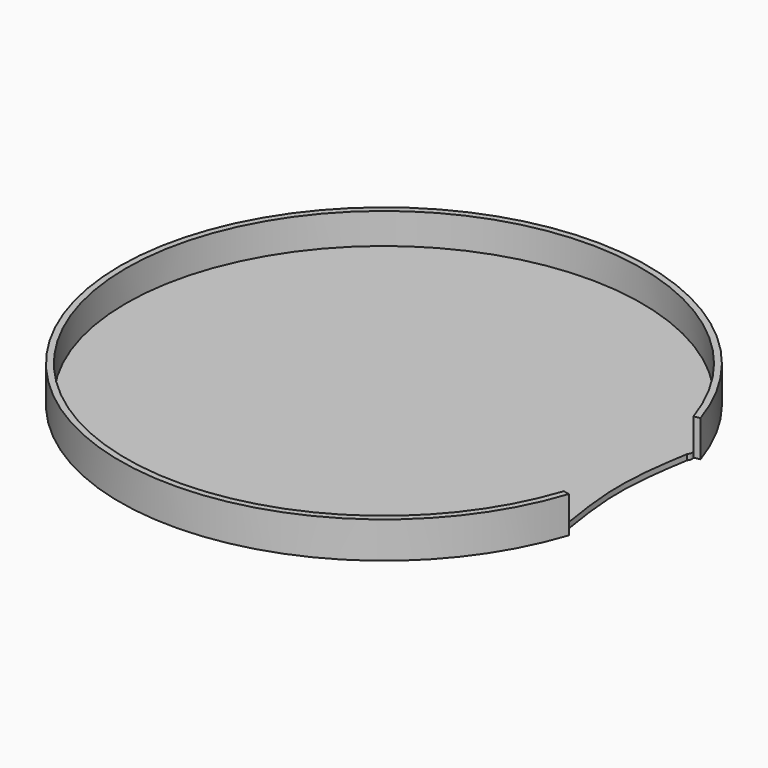
from build123d import *

# Parameters (mm, degrees)
F1_DEPTH    = 0.9
F2_DEPTH    = 5
F3_T1_DEPTH = 5.4053483188


# Not quite as in the source:
# - a fillet or chamfer that OpenCascade refuses, or shapes differently, is made with other operations: its cross-section is extruded or revolved along the edge and cut away or added


with BuildPart() as f1:
    # F0 (on Top) → F1 (new body)
    with BuildSketch(Plane.XY):
        with BuildLine():
            ThreePointArc((39.6825934579, 13.1351351897), (40.1749239484, 13.2423176115), (40.670911215, 13.3310532572))
            ThreePointArc((40.670911215, 13.3310532572), (-42.8, 0), (40.670911215, -13.3310532572))
            ThreePointArc((40.670911215, -13.3310532572), (40.1749239484, -13.2423176115), (39.6825934579, -13.1351351897))
            ThreePointArc((39.6825934579, -13.1351351897), (-41.8, 0), (39.6825934579, 13.1351351897))
        make_face()
        with BuildLine():
            ThreePointArc((39.5091459772, 12.0590331205), (39.7471474208, 12.1214723169), (39.9863317757, 12.179214717))
            ThreePointArc((39.9863317757, 12.179214717), (39.8373299552, 12.6580860339), (39.6825934579, 13.1351351897))
            add(Edge.make_bspline(
                [(39.5091459772, 12.0590331205), (39.5667025259, 12.4177338102), (39.6246479919, 12.7764345), (39.6825934579, 13.1351351897)],
                knots=[0.9590372671, 0.9590372671, 0.9590372671, 0.9590372671, 1, 1, 1, 1], degree=3))
        make_face()
        with BuildLine():
            ThreePointArc((39.6825934579, -13.1351351897), (39.8373299552, -12.6580860339), (39.9863317757, -12.179214717))
            ThreePointArc((39.9863317757, -12.179214717), (39.7471474208, -12.1214723169), (39.5091459772, -12.0590331205))
            add(Edge.make_bspline(
                [(39.6825934579, -13.1351351897), (39.6246479919, -12.7764345), (39.5667025259, -12.4177338102), (39.5091459772, -12.0590331205)],
                knots=[0, 0, 0, 0, 0.0409627329, 0.0409627329, 0.0409627329, 0.0409627329], degree=3))
        make_face()
        with BuildLine():
            add(Edge.make_bspline(
                [(39.5091459772, 12.0590331205), (39.5667025259, 12.4177338102), (39.6246479919, 12.7764345), (39.6825934579, 13.1351351897)],
                knots=[0.9590372671, 0.9590372671, 0.9590372671, 0.9590372671, 1, 1, 1, 1], degree=3))
            ThreePointArc((39.6825934579, 13.1351351897), (29.3, 0), (39.6825934579, -13.1351351897))
            add(Edge.make_bspline(
                [(39.6825934579, -13.1351351897), (39.6246479919, -12.7764345), (39.5667025259, -12.4177338102), (39.5091459772, -12.0590331205)],
                knots=[0, 0, 0, 0, 0.0409627329, 0.0409627329, 0.0409627329, 0.0409627329], degree=3))
            ThreePointArc((39.5091459772, -12.0590331205), (30.3, 0), (39.5091459772, 12.0590331205))
        make_face()
        with BuildLine():
            ThreePointArc((39.6825934579, -13.1351351897), (29.3, 0), (39.6825934579, 13.1351351897))
            ThreePointArc((39.6825934579, 13.1351351897), (-41.8, 0), (39.6825934579, -13.1351351897))
        make_face()
        with BuildLine():
            add(Edge.make_bspline(
                [(39.5091459772, -12.0590331205), (38.8641548126, -8.0393554137), (37.6718524129, 0), (38.8641548126, 8.0393554137), (39.5091459772, 12.0590331205)],
                knots=[0.0409627329, 0.0409627329, 0.0409627329, 0.0409627329, 0.5, 0.9590372671, 0.9590372671, 0.9590372671, 0.9590372671], degree=3))
            ThreePointArc((39.5091459772, 12.0590331205), (30.3, 0), (39.5091459772, -12.0590331205))
        make_face()
    extrude(amount=-F1_DEPTH)

    # F0 (on Top) → F2 (join)
    with BuildSketch(Plane.XY):
        with BuildLine():
            ThreePointArc((39.6825934579, 13.1351351897), (40.1749239484, 13.2423176115), (40.670911215, 13.3310532572))
            ThreePointArc((40.670911215, 13.3310532572), (-42.8, 0), (40.670911215, -13.3310532572))
            ThreePointArc((40.670911215, -13.3310532572), (40.1749239484, -13.2423176115), (39.6825934579, -13.1351351897))
            ThreePointArc((39.6825934579, -13.1351351897), (-41.8, 0), (39.6825934579, 13.1351351897))
        make_face()
    extrude(amount=F2_DEPTH)

    # F3: fillet of radius 1 on 2 edges, made by hand

    # F3_s2 → F3_t1 (cut)
    with BuildSketch(Plane.XY.offset(-3.1526741594)):
        with BuildLine():
            ThreePointArc((39.7145128215, -13.0383078407), (39.7431147732, -12.5211382035), (39.5091459772, -12.0590331205))
            ThreePointArc((39.5091459772, -12.0590331205), (39.7471474208, -12.1214723169), (39.9863317757, -12.179214717))
            ThreePointArc((39.9863317757, -12.179214717), (39.8527372664, -12.6094937398), (39.7145128215, -13.0383078407))
        make_face()
        with BuildLine():
            ThreePointArc((39.5091459772, 12.0590331205), (39.7431147732, 12.5211382035), (39.7145128215, 13.0383078407))
            ThreePointArc((39.7145128215, 13.0383078407), (39.8527372664, 12.6094937398), (39.9863317757, 12.179214717))
            ThreePointArc((39.9863317757, 12.179214717), (39.7471474208, 12.1214723169), (39.5091459772, 12.0590331205))
        make_face()
    extrude(amount=F3_T1_DEPTH, mode=Mode.SUBTRACT)


solid = f1.part
